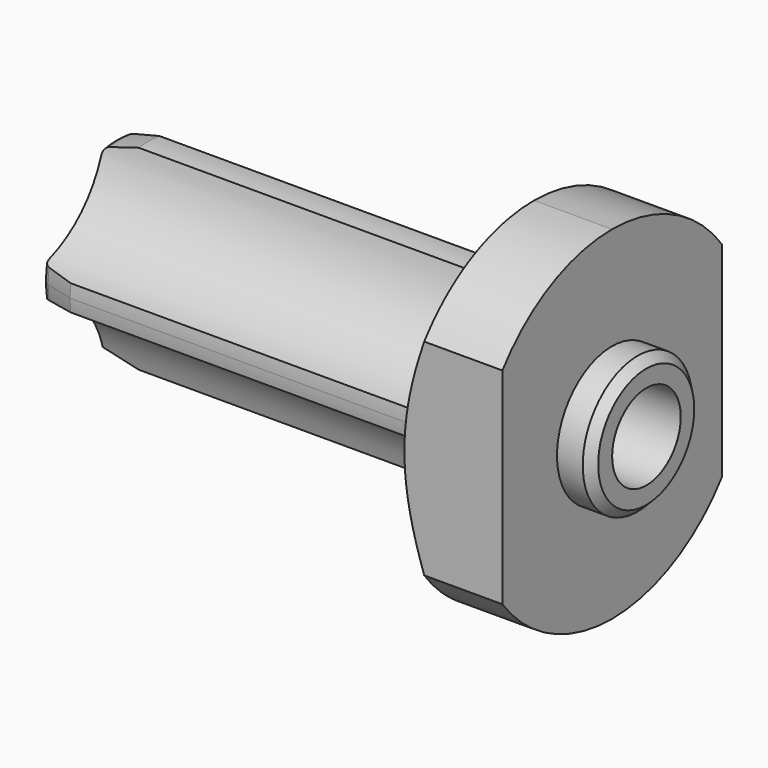
from build123d import *

# Parameters (mm, degrees)
F0_W      = 1.5
F0_H      = 1.5
F0_W_2    = 0.5
F0_H_2    = 0.435
F0_W_3    = 4.546262
F0_H_3    = 4
F0_H_4    = 2.065
F4_DEPTH  = 22
F5_SIZE2  = 2
F5_SIZE   = 0.5358983849
F6_R      = 0.5
F8_D      = 5
F8_DEPTH  = 10
F8_TIP    = 1.5021515476
F10_D     = 4
F10_DEPTH = 6
F10_TIP   = 1.2017212381
F12_DEPTH = 25


# Not quite as in the source:
# - ends of sketch curves that miss each other by under 0.0002 mm in the source are joined


with BuildPart() as f1:
    # F0 (on Top) → F1 (revolve)
    with BuildSketch(Plane.XY):
        with Locations((41.523095, 3.230684)):
            Rectangle(F0_W, F0_H)
        Polygon((33.773095, 5.681561), (33.773095, 2.480684), (37.5528260833, 2.480684), (36.226833, 5.980684), (36.226833, 9.980684), (33.773095, 5.730684), align=None)
        Polygon((36.226833, 5.980684), (37.5528260833, 2.480684), (39.4471019167, 2.480684), (40.773095, 5.980684), align=None)
        with Locations((42.523095, 2.263184)):
            Rectangle(F0_W_2, F0_H_2)
        Polygon((40.773095, 5.980684), (39.4471019167, 2.480684), (40.773095, 2.480684), (40.773095, 3.980684), align=None)
        with Locations((41.523095, 2.263184)):
            Rectangle(F0_W, F0_H_2)
        Polygon((42.273095, 3.980684), (42.273095, 2.480684), (42.773095, 2.480684), (42.773095, 3.480684), align=None)
        with Locations((38.499964, 7.980684)):
            Rectangle(F0_W_3, F0_H_3)
        with BuildLine():
            Line((40.773095, 2.045684), (40.773095, 0.7342315134))
            add(Edge.make_bspline(
                [(42.226833, -0.0193156), (42.2268322283, 0.4093938973), (40.773095, 0.7342315134)],
                knots=[3.141593, 3.141593, 3.141593, 3.8525916266, 3.8525916266, 3.8525916266], degree=2, weights=[1, 0.9374728154, 1]))
            Line((42.226833, -0.0193156), (42.273095, -0.019316))
            Line((42.273095, -0.019316), (42.273095, 2.045684))
            Line((42.273095, 2.045684), (40.773095, 2.045684))
        make_face()
        with Locations((42.523095, 1.013184)):
            Rectangle(F0_W_2, F0_H_4)
        Polygon((39.4471019167, 2.480684), (39.2822999192, 2.045684), (40.773095, 2.045684), (40.773095, 2.480684), align=None)
        with BuildLine():
            Line((33.773095, 0.730684), (33.773095, -0.019316))
            Line((33.773095, -0.019316), (34.273095, -0.019316))
            Line((34.273095, -0.019316), (38.499964, -0.019316))
            Line((38.499964, -0.019316), (38.0839828646, 1.0786791495))
            add(Edge.make_bspline(
                [(38.0839828646, 1.0786791495), (35.8841941746, 1.2164838646), (33.773095, 1.0344109623)],
                knots=[4.3976955436, 4.3976955436, 4.3976955436, 5.1336990724, 5.1336990724, 5.1336990724], degree=2, weights=[1, 0.9330480766, 1]))
            Line((33.773095, 1.0344109623), (33.773095, 0.730684))
        make_face()
        with BuildLine():
            Line((33.773095, 2.045684), (33.773095, 1.0344109623))
            add(Edge.make_bspline(
                [(38.0839828646, 1.0786791495), (35.8841941746, 1.2164838646), (33.773095, 1.0344109623)],
                knots=[4.3976955436, 4.3976955436, 4.3976955436, 5.1336990724, 5.1336990724, 5.1336990724], degree=2, weights=[1, 0.9330480766, 1]))
            Line((38.0839828646, 1.0786791495), (37.7176280808, 2.045684))
            Line((37.7176280808, 2.045684), (33.773095, 2.045684))
        make_face()
        Polygon((33.773095, 2.480684), (33.773095, 2.045684), (37.7176280808, 2.045684), (37.5528260833, 2.480684), align=None)
        with BuildLine():
            Line((37.7176280808, 2.045684), (38.0839828646, 1.0786791495))
            add(Edge.make_bspline(
                [(38.8919051119, 1.0152247595), (38.499964, 1.0526202094), (38.0839828646, 1.0786791495)],
                knots=[4.2521316371, 4.2521316371, 4.2521316371, 4.3976955436, 4.3976955436, 4.3976955436], degree=2, weights=[1, 0.9973525626, 1]))
            Line((38.8919051119, 1.0152247595), (39.2822999192, 2.045684))
            Line((39.2822999192, 2.045684), (37.7176280808, 2.045684))
        make_face()
        with BuildLine():
            Line((38.0839828646, 1.0786791495), (38.499964, -0.019316))
            Line((38.499964, -0.019316), (38.8919051119, 1.0152247595))
            add(Edge.make_bspline(
                [(38.8919051119, 1.0152247595), (38.499964, 1.0526202094), (38.0839828646, 1.0786791495)],
                knots=[4.2521316371, 4.2521316371, 4.2521316371, 4.3976955436, 4.3976955436, 4.3976955436], degree=2, weights=[1, 0.9973525626, 1]))
        make_face()
        with BuildLine():
            Line((38.8919051119, 1.0152247595), (38.499964, -0.019316))
            Line((38.499964, -0.019316), (40.773095, -0.019316))
            Line((40.773095, -0.019316), (40.773095, 0.7342315134))
            add(Edge.make_bspline(
                [(40.773095, 0.7342315134), (39.9803120127, 0.9113788897), (38.8919051119, 1.0152247595)],
                knots=[3.8525916266, 3.8525916266, 3.8525916266, 4.2521316371, 4.2521316371, 4.2521316371], degree=2, weights=[1, 0.9801122448, 1]))
        make_face()
        Polygon((37.5528260833, 2.480684), (37.7176280808, 2.045684), (39.2822999192, 2.045684), (39.4471019167, 2.480684), align=None)
        with BuildLine():
            Line((39.2822999192, 2.045684), (38.8919051119, 1.0152247595))
            add(Edge.make_bspline(
                [(40.773095, 0.7342315134), (39.9803120127, 0.9113788897), (38.8919051119, 1.0152247595)],
                knots=[3.8525916266, 3.8525916266, 3.8525916266, 4.2521316371, 4.2521316371, 4.2521316371], degree=2, weights=[1, 0.9801122448, 1]))
            Line((40.773095, 0.7342315134), (40.773095, 2.045684))
            Line((40.773095, 2.045684), (39.2822999192, 2.045684))
        make_face()
        with BuildLine():
            Line((40.773095, 0.7342315134), (40.773095, -0.019316))
            Line((40.773095, -0.019316), (42.226833, -0.019316))
            add(Edge.make_bspline(
                [(42.226833, -0.019316), (42.2268322283, 0.4093938973), (40.773095, 0.7342315134)],
                knots=[3.141593, 3.141593, 3.141593, 3.8525916266, 3.8525916266, 3.8525916266], degree=2, weights=[1, 0.9374728154, 1]))
        make_face()
    revolve(axis=Axis((20.5738751867, -0.019316, 0), (1, 0, 0)))

    # F3 (on face) → F4 (join)
    with BuildSketch(Plane(origin=(33.773095, 0, 0), x_dir=(0, -1, 0), z_dir=(-1, 0, 0))):
        with BuildLine():
            ThreePointArc((0.7512693785, 5.7032222692), (-0.000602262, 5.749965501), (-0.7521320187, 5.698014387))
            ThreePointArc((-0.7521320187, 5.698014387), (-2.4254688054, 2.4414028529), (-5.6797608355, 0.7635595739))
            ThreePointArc((-5.6797608355, 0.7635595739), (-5.7306746348, 0.0103778617), (-5.6824799161, -0.7429827264))
            ThreePointArc((-5.6824799161, -0.7429827264), (-2.4218166649, -2.4249412056), (-0.7499999869, -5.6908159978))
            ThreePointArc((-0.7499999869, -5.6908159978), (0, -5.739939), (0.7500000036, -5.690816125))
            ThreePointArc((0.7500000036, -5.690816125), (2.4284043129, -2.4183433129), (5.7008769978, -0.7399389869))
            ThreePointArc((5.7008769978, -0.7399389869), (5.7377061387, -0.3657424933), (5.75, 0.010061))
            ThreePointArc((5.75, 0.010061), (5.7377061387, 0.3858644933), (5.700877125, 0.7600610036))
            ThreePointArc((5.700877125, 0.7600610036), (2.4311698073, 2.43570162), (0.7512693785, 5.7032222692))
        make_face()
    extrude(amount=F4_DEPTH)

    # F5
    f5_edges = [f1.edges().sort_by_distance(p)[0] for p in [
        (11.773095, 0.000602, 5.749966),
        (11.773095, -5.737706, 0.385864),
        (11.773095, 0, -5.739939),
        (11.773095, 5.730675, 0.010378),
    ]]
    f5_side = f1.faces().sort_by_distance((11.773095, -0.002803, 0.008597))[0]
    chamfer(f5_edges, length=F5_SIZE, length2=F5_SIZE2, reference=f5_side)

    # F6
    f6_edges = [f1.edges().sort_by_distance(p)[0] for p in [
        (11.773095, 0.001201, 5.214061),
        (11.773095, 5.194775, 0.010692),
        (11.773095, -5.195822, 0.446281),
    ]]
    fillet(f6_edges, radius=F6_R)

    # F8
    with Locations(Plane.YZ.offset(42.773095)):
        with Locations((0, 0)):
            Hole(F8_D / 2, depth=F8_DEPTH)
            with Locations((0, 0, -(F8_DEPTH + F8_TIP / 2))):  # 118° drill point
                Cone(0, F8_D / 2, F8_TIP, mode=Mode.SUBTRACT)

    # F10
    with Locations(Plane(origin=(11.773095, 0, 0), x_dir=(0, -1, 0), z_dir=(-1, 0, 0))):
        with Locations((0, 0)):
            Hole(F10_D / 2, depth=F10_DEPTH)
            with Locations((0, 0, -(F10_DEPTH + F10_TIP / 2))):  # 118° drill point
                Cone(0, F10_D / 2, F10_TIP, mode=Mode.SUBTRACT)

    # F11 (on face) → F12 (cut)
    with BuildSketch(Plane.YZ.offset(40.773095)):
        with BuildLine():
            ThreePointArc((8, -5.9741585928), (9.4726058286, -3.1469699713), (9.980684, 0))
            ThreePointArc((9.980684, 0), (9.4726058286, 3.1469699713), (8, 5.9741585928))
            Line((8, 5.9741585928), (8, -5.9741585928))
        make_face()
        with BuildLine():
            ThreePointArc((-8, 6), (-4.476454623, 8.9421112724), (-0.009658, 9.9999953362))
            ThreePointArc((-0.009658, 9.9999953362), (-10.019316, 0), (-0.009658, -9.9999953362))
            ThreePointArc((-0.009658, -9.9999953362), (-4.476454623, -8.9421112724), (-8, -6))
            Line((-8, -6), (-8, 6))
        make_face()
    extrude(amount=-F12_DEPTH, mode=Mode.SUBTRACT)


solid = f1.part
